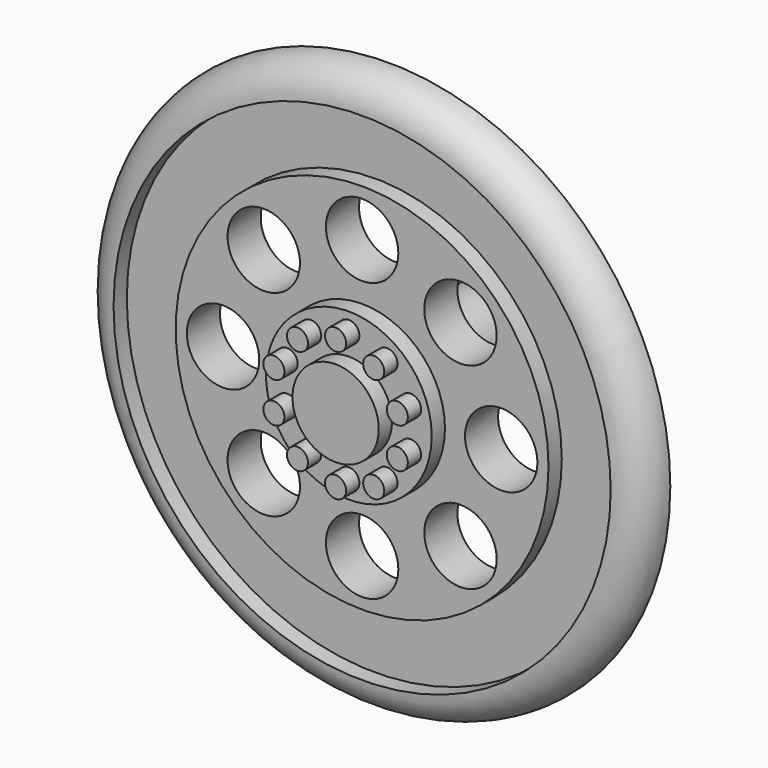
from build123d import *

# Parameters (mm, degrees)
F0_R      = 17
F1_DEPTH  = 2.5
F2_R      = 2
F4_R      = 15
F4_R_2    = 11.25
F6_DEPTH  = 1
F5_R      = 5
F8_DEPTH  = 1
F7_R      = 2.1850910156
F9_DEPTH  = 25.4
F10_R     = 2.6038843179
F11_DEPTH = 1
F12_R     = 0.6358860885
F13_DEPTH = 0.5
F14_DEPTH = 0.5
F15_R     = 2.3875943528
F16_DEPTH = 7.5


# Not quite as in the source:
# - a fillet or chamfer that OpenCascade refuses, or shapes differently, is made with other operations: its cross-section is extruded or revolved along the edge and cut away or added


with BuildPart() as f1:
    # F0 (on Front) → F1 (new body)
    with BuildSketch(Plane.XZ):
        Circle(F0_R)
    extrude(amount=F1_DEPTH)

    # F2
    f2_edges = [f1.edges().sort_by_distance(p)[0] for p in [
        (-17, -2.5, 0),
    ]]
    fillet(f2_edges, radius=F2_R)

    # F3: fillet of radius 2 on 1 edges, made by hand

    # F3_s1 → F3_t2 (revolve, cut)
    with BuildSketch(Plane.XY):
        with BuildLine():
            ThreePointArc((17, -0.5), (16.3842311257, -0.1291713066), (15.6771243445, 0))
            Line((15.6771243445, 0), (17, 0))
            Line((17, 0), (17, -0.5))
        make_face()
    revolve(axis=Axis((0, 0, 0), (0, -1, 0)), mode=Mode.SUBTRACT)

    # F4 (on face) → F6 (cut)
    with BuildSketch(Plane.XZ.offset(2.5)):
        Circle(F4_R)
        Circle(F4_R_2, mode=Mode.SUBTRACT)
    extrude(amount=-F6_DEPTH, mode=Mode.SUBTRACT)

    # F5 (on face) → F8 (join)
    with BuildSketch(Plane.XZ.offset(2.5)):
        Circle(F5_R)
    extrude(amount=F8_DEPTH)

    # F7 (on face) → F9 (cut)
    with BuildSketch(Plane.XZ.offset(2.5)):
        with Locations((0, 8.3935074508)):
            Circle(F7_R)
        with Locations((5.9351060364, 5.9351060364)):
            Circle(F7_R)
        with Locations((8.3935074508, 0)):
            Circle(F7_R)
        with Locations((5.9351060364, -5.9351060364)):
            Circle(F7_R)
        with Locations((0, -8.3935074508)):
            Circle(F7_R)
        with Locations((-5.9351060364, -5.9351060364)):
            Circle(F7_R)
        with Locations((-8.3935074508, 0)):
            Circle(F7_R)
        with Locations((-5.9351060364, 5.9351060364)):
            Circle(F7_R)
    extrude(amount=-F9_DEPTH, mode=Mode.SUBTRACT)

    # F10 (on face) → F11 (join)
    with BuildSketch(Plane.XZ.offset(3.5)):
        Circle(F10_R)
    extrude(amount=F11_DEPTH)

    # F12 (on face) → F13 (join)
    with BuildSketch(Plane.XZ.offset(3.5)):
        with Locations((-2.3013945397, 3.1675978363)):
            Circle(F12_R)
        with Locations((0, 3.915366251)):
            Circle(F12_R)
        with Locations((2.3013945397, 3.1675978363)):
            Circle(F12_R)
        with Locations((3.7237345867, 1.2099147108)):
            Circle(F12_R)
        with Locations((3.7237345867, -1.2099147108)):
            Circle(F12_R)
        with Locations((2.3013945397, -3.1675978363)):
            Circle(F12_R)
        with Locations((0, -3.915366251)):
            Circle(F12_R)
        with Locations((-2.3013945397, -3.1675978363)):
            Circle(F12_R)
        with Locations((-3.7237345867, -1.2099147108)):
            Circle(F12_R)
        with Locations((-3.7237345867, 1.2099147108)):
            Circle(F12_R)
    extrude(amount=F13_DEPTH)

    # F14 (add): faces of the model
    f14_faces = [f1.faces().sort_by_distance(p)[0] for p in [
        (3.7237345867, -4, 1.2099147108),
        (2.3013945397, -4, 3.1675978363),
        (0, -4, 3.915366251),
        (-2.3013945397, -4, 3.1675978363),
        (-3.7237345867, -4, 1.2099147108),
        (-3.7237345867, -4, -1.2099147108),
        (-2.3013945397, -4, -3.1675978363),
        (0, -4, -3.915366251),
        (2.3013945397, -4, -3.1675978363),
        (3.7237345867, -4, -1.2099147108),
    ]]
    extrude(f14_faces, amount=F14_DEPTH)

    # F15 (on face) → F16 (join)
    with BuildSketch(Plane(origin=(0, 0, 0), x_dir=(-1, 0, 0), z_dir=(0, 1, 0))):
        Circle(F15_R)
    extrude(amount=F16_DEPTH)


solid = f1.part
